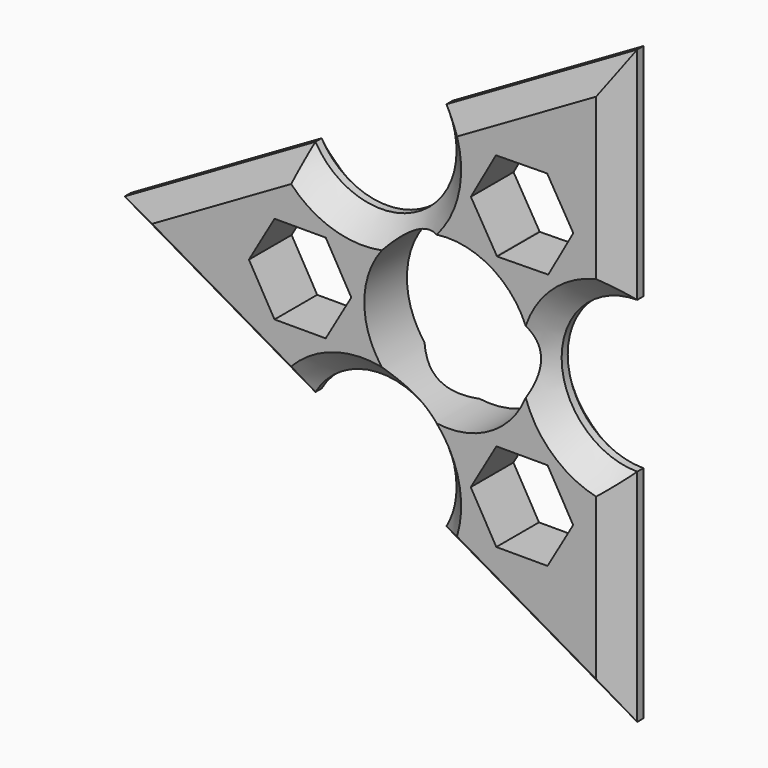
from build123d import *

# Parameters (mm, degrees)
F0_R         = 11
F1_DEPTH     = 7
F2_T1_DEPTH  = 44.3442261521
F2_T3_DEPTH  = 44.3442261521
F2_T5_DEPTH  = 44.3442261521
F2_T7_DEPTH  = 44.3442261521
F2_T9_DEPTH  = 44.3442261521
F2_T11_DEPTH = 44.3442261521
F2_T14_ANGLE = 269.2452016921
F2_T16_ANGLE = 269.2452016921
F2_T18_ANGLE = 269.2452016921
F2_T20_ANGLE = 269.2452016921
F2_T22_ANGLE = 269.2452016921
F2_T24_ANGLE = 269.2452016921
F4_DEPTH     = 25.4
F5_DEPTH     = 25.4


# Not quite as in the source:
# - a fillet or chamfer that OpenCascade refuses, or shapes differently, is made with other operations: its cross-section is extruded or revolved along the edge and cut away or added
# - a feature names something its author has since deleted; it is built from what else it names


with BuildPart() as f1:
    # F0 (on Front) → F1 (new body)
    with BuildSketch(Plane.XZ):
        with BuildLine():
            Line((-19.8038627003, 14.4570641122), (-44.8442322709, 0))
            Line((-44.8442322709, 0), (-19.8038627003, -14.4570641122))
            ThreePointArc((-19.8038627003, -14.4570641122), (-8.6430254441, -9.8340939532), (-1.2889419323, -19.4181221799))
            ThreePointArc((-1.2889419323, -19.4181221799), (-1.6270298411, -21.9861548035), (-2.6182534351, -24.3791802476))
            Line((-2.6182534351, -24.3791802476), (22.4221161354, -38.8362443598))
            Line((22.4221161354, -38.8362443598), (22.4221161354, -9.9221161354))
            ThreePointArc((22.4221161354, -9.9221161354), (12.5, 0), (22.4221161354, 9.9221161354))
            Line((22.4221161354, 9.9221161354), (22.4221161354, 38.8362443598))
            Line((22.4221161354, 38.8362443598), (-2.6182534351, 24.3791802476))
            ThreePointArc((-2.6182534351, 24.3791802476), (-1.6270298411, 21.9861548035), (-1.2889419323, 19.4181221799))
            ThreePointArc((-1.2889419323, 19.4181221799), (-8.6430254441, 9.8340939532), (-19.8038627003, 14.4570641122))
        make_face()
        Circle(F0_R, mode=Mode.SUBTRACT)
    extrude(amount=-F1_DEPTH)

    # F2: chamfer of 3 on 18 edges, made by hand

    # F2_s2 → F2_t1 (cut)
    with BuildSketch(Plane(origin=(40.3146025973, 0, 23.2756466618), x_dir=(0, 1, 0), z_dir=(-0.8660254038, 0, -0.5))):
        Polygon((7, -19.4221161354), (4, -22.4221161354), (7, -22.4221161354), align=None)
        Polygon((3, -22.4221161354), (0, -19.4221161354), (0, -22.4221161354), align=None)
    extrude(amount=F2_T1_DEPTH, mode=Mode.SUBTRACT)

    # F2_s4 → F2_t3 (cut)
    with BuildSketch(Plane(origin=(-1.9113762384, 0, -1.1035335858), x_dir=(0, 1, 0), z_dir=(-0.8660254038, 0, -0.5))):
        Polygon((3, -22.4221161354), (0, -19.4221161354), (0, -22.4221161354), align=None)
        Polygon((4, -22.4221161354), (7, -19.4221161354), (7, -22.4221161354), align=None)
    extrude(amount=F2_T3_DEPTH, mode=Mode.SUBTRACT)

    # F2_s6 → F2_t5 (cut)
    with BuildSketch(Plane(origin=(-40.3146025973, 0, 23.2756466618), x_dir=(0, 1, 0), z_dir=(0.8660254038, 0, -0.5))):
        Polygon((0, -19.4221161354), (3, -22.4221161354), (0, -22.4221161354), align=None)
        Polygon((7, -19.4221161354), (4, -22.4221161354), (7, -22.4221161354), align=None)
    extrude(amount=F2_T5_DEPTH, mode=Mode.SUBTRACT)

    # F2_s8 → F2_t7 (cut)
    with BuildSketch(Plane(origin=(1.9113762384, 0, -1.1035335858), x_dir=(0, 1, 0), z_dir=(0.8660254038, 0, -0.5))):
        Polygon((3, -22.4221161354), (0, -19.4221161354), (0, -22.4221161354), align=None)
        Polygon((7, -19.4221161354), (4, -22.4221161354), (7, -22.4221161354), align=None)
    extrude(amount=F2_T7_DEPTH, mode=Mode.SUBTRACT)

    # F2_s10 → F2_t9 (cut)
    with BuildSketch(Plane.XY.offset(-46.5512933237)):
        Polygon((22.4221161354, 3), (19.4221161354, 0), (22.4221161354, 0), align=None)
        Polygon((19.4221161354, 7), (22.4221161354, 4), (22.4221161354, 7), align=None)
    extrude(amount=F2_T9_DEPTH, mode=Mode.SUBTRACT)

    # F2_s12 → F2_t11 (cut)
    with BuildSketch(Plane.XY.offset(2.2070671715)):
        Polygon((22.4221161354, 3), (19.4221161354, 0), (22.4221161354, 0), align=None)
        Polygon((19.4221161354, 7), (22.4221161354, 4), (22.4221161354, 7), align=None)
    extrude(amount=F2_T11_DEPTH, mode=Mode.SUBTRACT)

    # F2_s13 → F2_t14 (revolve, cut)
    with BuildSketch(Plane(origin=(4.0288460704, 0, 15.4420044307), x_dir=(0, 1, 0), z_dir=(0.2524510604, 0, 0.9676096641))):
        Polygon((0, 28.6721698019), (3, 25.6721698019), (0, 25.6721698019), align=None)
    revolve(axis=Axis((-11.2110580677, 0, 19.4181221799), (0, -1, 0)), revolution_arc=F2_T14_ANGLE, mode=Mode.SUBTRACT)

    # F2_s15 → F2_t16 (revolve, cut)
    with BuildSketch(Plane(origin=(-15.3875911575, 0, 4.2319191704), x_dir=(0, 1, 0), z_dir=(-0.9642000803, 0, 0.2651758006))):
        Polygon((7, -28.6721698019), (4, -25.6721698019), (7, -25.6721698019), align=None)
    revolve(axis=Axis((-11.2110580677, 7, 19.4181221799), (0, 1, 0)), revolution_arc=F2_T16_ANGLE, mode=Mode.SUBTRACT)

    # F2_s17 → F2_t18 (revolve, cut)
    with BuildSketch(Plane(origin=(-15.3875911575, 0, -4.2319191704), x_dir=(0, 1, 0), z_dir=(-0.9642000803, 0, -0.2651758006))):
        Polygon((3, 25.6721698019), (0, 28.6721698019), (0, 25.6721698019), align=None)
    revolve(axis=Axis((-11.2110580677, 0, -19.4181221799), (0, -1, 0)), revolution_arc=F2_T18_ANGLE, mode=Mode.SUBTRACT)

    # F2_s19 → F2_t20 (revolve, cut)
    with BuildSketch(Plane(origin=(4.0288460704, 0, -15.4420044307), x_dir=(0, 1, 0), z_dir=(0.2524510604, 0, -0.9676096641))):
        Polygon((7, -28.6721698019), (4, -25.6721698019), (7, -25.6721698019), align=None)
    revolve(axis=Axis((-11.2110580677, 7, -19.4181221799), (0, 1, 0)), revolution_arc=F2_T20_ANGLE, mode=Mode.SUBTRACT)

    # F2_s21 → F2_t22 (revolve, cut)
    with BuildSketch(Plane(origin=(11.3587450871, 0, 11.2100852602), x_dir=(0, 1, 0), z_dir=(0.7117490199, 0, 0.7024338636))):
        Polygon((3, -25.6721698019), (0, -28.6721698019), (0, -25.6721698019), align=None)
    revolve(axis=Axis((22.4221161354, 0, 0), (0, 1, 0)), revolution_arc=F2_T22_ANGLE, mode=Mode.SUBTRACT)

    # F2_s23 → F2_t24 (revolve, cut)
    with BuildSketch(Plane(origin=(11.3587450871, 0, 11.2100852602), x_dir=(0, 1, 0), z_dir=(0.7117490199, 0, 0.7024338636))):
        Polygon((7, -28.6721698019), (4, -25.6721698019), (7, -25.6721698019), align=None)
    revolve(axis=Axis((22.4221161354, 7, 0), (0, 1, 0)), revolution_arc=F2_T24_ANGLE, mode=Mode.SUBTRACT)

    # F3 (on face) → F4 (cut)
    with BuildSketch(Plane.XZ):
        Polygon((13.0480463402, 22.5998792008), (6.3740697952, 11.0402127363), (6.4247100072, 10.9550491246), (13.1471202974, 11.0414866405), (16.4334683579, 16.9064834844), align=None)
        Polygon((2.9886477775, 16.7336084526), (6.3740697952, 11.0402127363), (13.0480463402, 22.5998792008), (12.9974061282, 22.6850428125), (6.274995838, 22.5986052966), align=None)
        Polygon((-26.1366, 0), (-12.7, 0), (-16.05915, 5.8182184702), (-22.77745, 5.8182184702), align=None)
        Polygon((-16.05915, -5.8182184702), (-12.7, 0), (-26.1366, 0), (-22.77745, -5.8182184702), align=None)
    extrude(amount=-F4_DEPTH, mode=Mode.SUBTRACT)

    # F3 (on face) → F5 (cut)
    with BuildSketch(Plane.XZ):
        Polygon((2.9886477775, 16.7336084526), (6.3740697952, 11.0402127363), (13.0480463402, 22.5998792008), (12.9974061282, 22.6850428125), (6.274995838, 22.5986052966), align=None)
        Polygon((13.0480463402, 22.5998792008), (6.3740697952, 11.0402127363), (6.4247100072, 10.9550491246), (13.1471202974, 11.0414866405), (16.4334683579, 16.9064834844), align=None)
        Polygon((-16.05915, -5.8182184702), (-12.7, 0), (-26.1366, 0), (-22.77745, -5.8182184702), align=None)
        Polygon((-26.1366, 0), (-12.7, 0), (-16.05915, 5.8182184702), (-22.77745, 5.8182184702), align=None)
        Polygon((13.0581752927, -11.0105414452), (6.3398781361, -11.0043602821), (13.0474692042, -22.6469734606), (16.4119708267, -16.8318480344), align=None)
        Polygon((13.0474692042, -22.6469734606), (6.3398781361, -11.0043602821), (2.9753765137, -16.8194857083), (6.3291720477, -22.6407922976), align=None)
    extrude(amount=-F5_DEPTH, mode=Mode.SUBTRACT)


solid = f1.part
